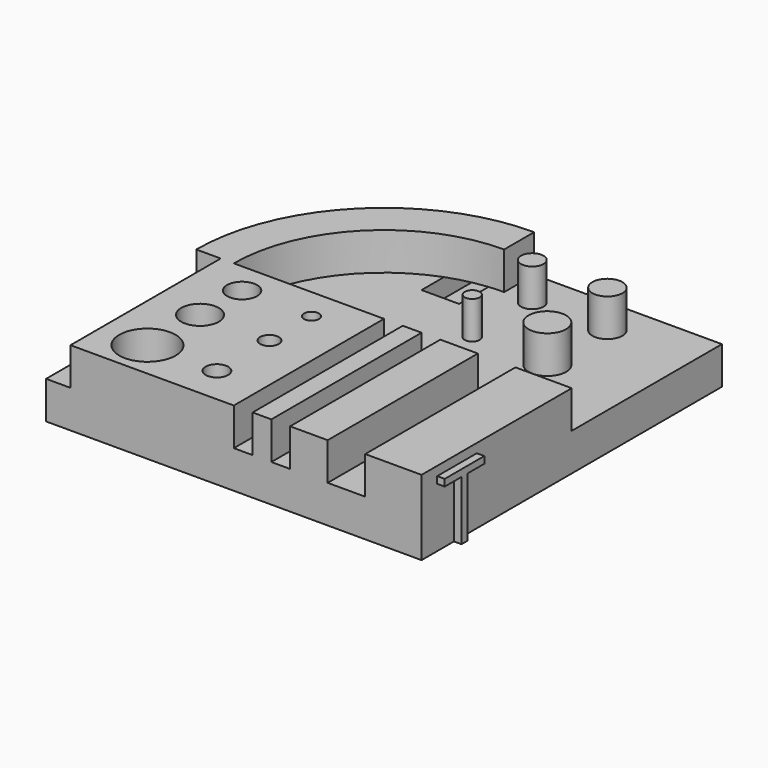
from build123d import *

# Parameters (mm, degrees)
F1_DEPTH     = 2
F2_W         = 8.7
F2_H         = 10
F2_R         = 1.5
F2_R_2       = 0.6
F2_R_3       = 1
F2_R_4       = 0.8
F2_R_5       = 0.5
F2_R_6       = 0.4
F2_W_2       = 3
F2_W_3       = 2
F2_W_4       = 1
F3_DEPTH     = 2
F4_W         = 2
F4_H         = 2
F5_ANGLE     = 90
F7_DEPTH     = 1
F8_TEXT_SIZE = 4.9281314168
F9_DEPTH     = 0.4


# Not quite as in the source:
# - Text() gives the source's letters only with a copy of the font that has no kerning and outlines rounded to 1/6400 em; it was checked with that copy


with BuildPart() as f1:
    # F0 (on Top) → F1 (new body)
    with BuildSketch(Plane.XY):
        with BuildLine():
            Line((-10, -10), (10, -10))
            Line((10, -10), (10, 10))
            Line((10, 10), (0, 10))
            ThreePointArc((0, 10), (-7.0710678119, 7.0710678119), (-10, 0))
            Line((-10, 0), (-10, -10))
        make_face()
    extrude(amount=F1_DEPTH)

    # F2 (on face) → F3 (join)
    with BuildSketch(Plane.XY.offset(2)):
        with Locations((-4.35, -5)):
            Rectangle(F2_W, F2_H)
        with Locations((-6.2, -8)):
            Circle(F2_R, mode=Mode.SUBTRACT)
        with Locations((-2.5, -8)):
            Circle(F2_R_2, mode=Mode.SUBTRACT)
        with Locations((-6.2, -4.5)):
            Circle(F2_R_3, mode=Mode.SUBTRACT)
        with Locations((-6.2, -1.7)):
            Circle(F2_R_4, mode=Mode.SUBTRACT)
        with Locations((-2.5, -4.5)):
            Circle(F2_R_5, mode=Mode.SUBTRACT)
        with Locations((-2.5, -1.7)):
            Circle(F2_R_6, mode=Mode.SUBTRACT)
        with Locations((8.5, -5)):
            Rectangle(F2_W_2, F2_H)
        with Locations((4, -5)):
            Rectangle(F2_W_3, F2_H)
        with Locations((1.5, -5)):
            Rectangle(F2_W_4, F2_H)
        with Locations((1.5, 4)):
            Circle(F2_R_6)
        with Locations((5.5, 4)):
            Circle(F2_R_3)
        with Locations((5.5, 8)):
            Circle(F2_R_4)
        with Locations((1.5, 8)):
            Circle(F2_R_2)
    extrude(amount=F3_DEPTH)

    # F4 (on Right) → F5 (revolve)
    with BuildSketch(Plane.YZ):
        with Locations((9, 3)):
            Rectangle(F4_W, F4_H)
    revolve(axis=Axis((0, 0, 6.4536398277), (0, 0, 1)), revolution_arc=F5_ANGLE)

    # F6 (on face) → F7 (cut)
    with BuildSketch(Plane.XY.offset(2)):
        with BuildLine():
            ThreePointArc((-7.9598994969, 0.8), (-7.7913884421, 1.8150113346), (-7.4939975981, 2.8))
            Line((-7.4939975981, 2.8), (-10, 2.8))
            Line((-10, 2.8), (-10, 0.8))
            Line((-10, 0.8), (-7.9598994969, 0.8))
        make_face()
        with BuildLine():
            Line((-0.8, 7.9598994969), (-0.8, 10))
            Line((-0.8, 10), (-2.8, 10))
            Line((-2.8, 10), (-2.8, 7.4939975981))
            ThreePointArc((-2.8, 7.4939975981), (-1.8150113346, 7.7913884421), (-0.8, 7.9598994969))
        make_face()
        with BuildLine():
            Line((-6, 2.8), (-7.4939975981, 2.8))
            ThreePointArc((-7.4939975981, 2.8), (-7.7913884421, 1.8150113346), (-7.9598994969, 0.8))
            Line((-7.9598994969, 0.8), (-6, 0.8))
            Line((-6, 0.8), (-6, 2.8))
        make_face()
        with BuildLine():
            Line((-0.8, 6), (-0.8, 7.9598994969))
            ThreePointArc((-0.8, 7.9598994969), (-1.8150113346, 7.7913884421), (-2.8, 7.4939975981))
            Line((-2.8, 7.4939975981), (-2.8, 6))
            Line((-2.8, 6), (-0.8, 6))
        make_face()
    extrude(amount=-F7_DEPTH, mode=Mode.SUBTRACT)

    # F8 (on face) → F9 (join)
    with BuildSketch(Plane.YZ.offset(10)):
        with Locations((-9, 0)):
            Text('T', F8_TEXT_SIZE, font='Open Sans', text_align=(TextAlign.LEFT, TextAlign.BOTTOM))
    extrude(amount=F9_DEPTH)


solid = f1.part
